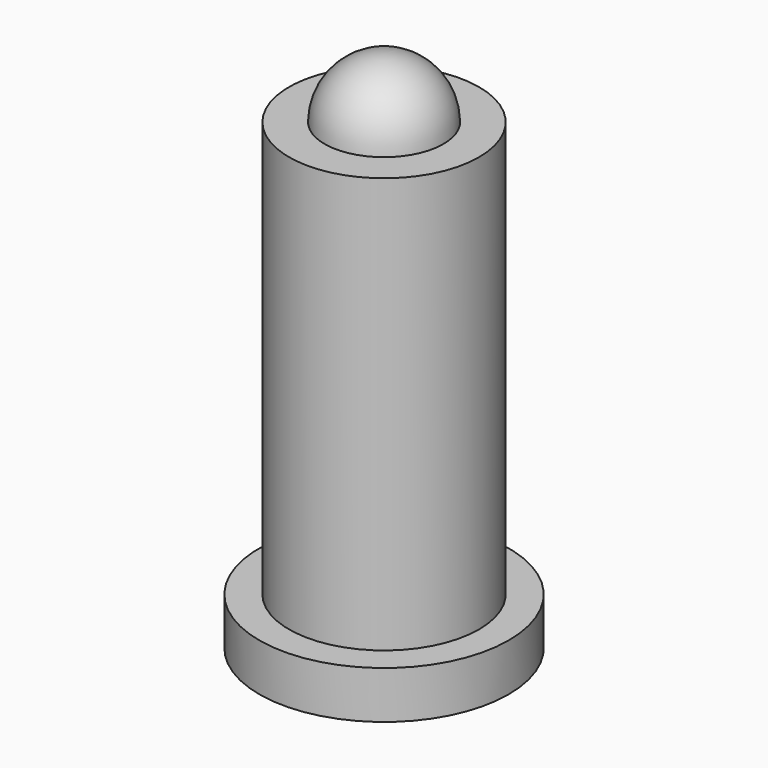
from build123d import *

# Parameters (mm, degrees)
F0_R     = 10.5
F1_DEPTH = 4
F2_R     = 8
F3_DEPTH = 39


# Not quite as in the source:
# - a feature names something its author has since deleted; it is built from what else it names


with BuildPart() as f1:
    # F0 (on Top) → F1 (new body)
    with BuildSketch(Plane.XY):
        Circle(F0_R)
    extrude(amount=F1_DEPTH)

    # F2 (on Top) → F3 (join)
    with BuildSketch(Plane.XY):
        Circle(F2_R)
    extrude(amount=F3_DEPTH)

    # F4 (on Right) → F5 (revolve)
    with BuildSketch(Plane.YZ):
        with BuildLine():
            ThreePointArc((5, 39), (3.5355339059, 42.5355339059), (0, 44))
            Line((0, 44), (0, 39))
            Line((0, 39), (5, 39))
        make_face()
    revolve(axis=Axis((0, 0, 41.5), (0, 0, -1)))


solid = f1.part
